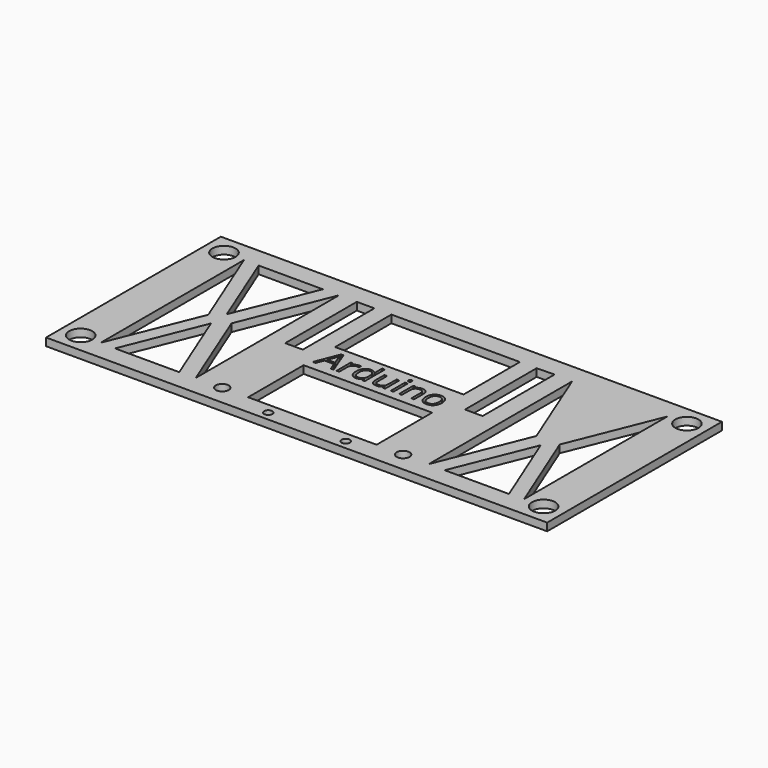
from build123d import *

# Parameters (mm, degrees)
F0_W         = 247.65
F0_H         = 107.95
F0_R         = 5.715
F0_R_2       = 3.175
F0_R_3       = 2.032
F0_W_2       = 63.5
F0_H_2       = 34.3049401417
F0_W_3       = 8.6955651641
F0_H_3       = 44.2145633824
F0_H_4       = 34.7810434178
F1_DEPTH     = 3.81
F2_TEXT_SIZE = 16.3904158399
F3_DEPTH     = 2.032


# Not quite as in the source:
# - ends of sketch curves that miss each other by under 0.0002 mm in the source are joined
# - Text() gives the source's letters only with a copy of the font that has no kerning and outlines rounded to 1/6400 em; it was checked with that copy


with BuildPart() as f1:
    # F0 (on Top) → F1 (new body)
    with BuildSketch(Plane.XY):
        Rectangle(F0_W, F0_H)
        with Locations((-114.4934743643, -44.2593507469)):
            Circle(F0_R, mode=Mode.SUBTRACT)
        with Locations((-44.5289053023, -44.2593507469)):
            Circle(F0_R_2, mode=Mode.SUBTRACT)
        with Locations((-17.6647994667, -49.421813339)):
            Circle(F0_R_3, mode=Mode.SUBTRACT)
        Polygon((-65.6054269843, -44.4832319825), (-97.3554269843, -44.4832319825), (-81.4804269843, -5.0392397434), align=None, mode=Mode.SUBTRACT)
        Polygon((-75.3409461476, -0.0447873644), (-57.6003963857, 44.2145633824), (-57.6003963857, -44.3041381113), align=None, mode=Mode.SUBTRACT)
        with Locations((20.6495840102, -49.421813339)):
            Circle(F0_R_3, mode=Mode.SUBTRACT)
        with Locations((44.8713228106, -44.3041381113)):
            Circle(F0_R_2, mode=Mode.SUBTRACT)
        with Locations((0, -27.106880676)):
            Rectangle(F0_W_2, F0_H_2, mode=Mode.SUBTRACT)
        with Locations((114.2910420895, -44.2593507469)):
            Circle(F0_R, mode=Mode.SUBTRACT)
        Polygon((97.3554269843, -44.4832319825), (65.6054269843, -44.4832319825), (81.4804269843, -5.0392397434), align=None, mode=Mode.SUBTRACT)
        Polygon((57.6003963857, -44.3041381113), (57.6003963857, 44.2145633824), (75.3409461476, -0.0447873644), align=None, mode=Mode.SUBTRACT)
        Polygon((86.8265612391, 0), (104.6215225417, 44.2144450718), (104.6395568408, -44.2593507548), align=None, mode=Mode.SUBTRACT)
        Polygon((-104.639595702, -44.2593507469), (-104.639595702, 44.2593507469), (-86.8265612391, 0), align=None, mode=Mode.SUBTRACT)
        Polygon((-97.3554269843, 44.2593507469), (-65.6054269843, 44.2145633824), (-81.5360676272, 4.7930104264), align=None, mode=Mode.SUBTRACT)
        with Locations((-44.4727316499, 22.1072816912)):
            Rectangle(F0_W_3, F0_H_3, mode=Mode.SUBTRACT)
        with Locations((-114.4934743643, 44.2593507469)):
            Circle(F0_R, mode=Mode.SUBTRACT)
        with Locations((0, 26.868829038)):
            Rectangle(F0_W_2, F0_H_4, mode=Mode.SUBTRACT)
        Polygon((40.026973933, 0), (40.026973933, 44.2593507469), (48.722536933, 44.45), (48.722536933, 0), align=None, mode=Mode.SUBTRACT)
        with Locations((114.2910420895, 44.2593507469)):
            Circle(F0_R, mode=Mode.SUBTRACT)
    extrude(amount=F1_DEPTH)

    # F2 (on face) → F3 (cut)
    with BuildSketch(Plane.XY.offset(3.81)):
        with Locations((-30.7077001762, -5.6415549479)):
            Text('Arduino', F2_TEXT_SIZE, font='Open Sans', text_align=(TextAlign.LEFT, TextAlign.BOTTOM))
    extrude(amount=-F3_DEPTH, mode=Mode.SUBTRACT)


solid = f1.part
